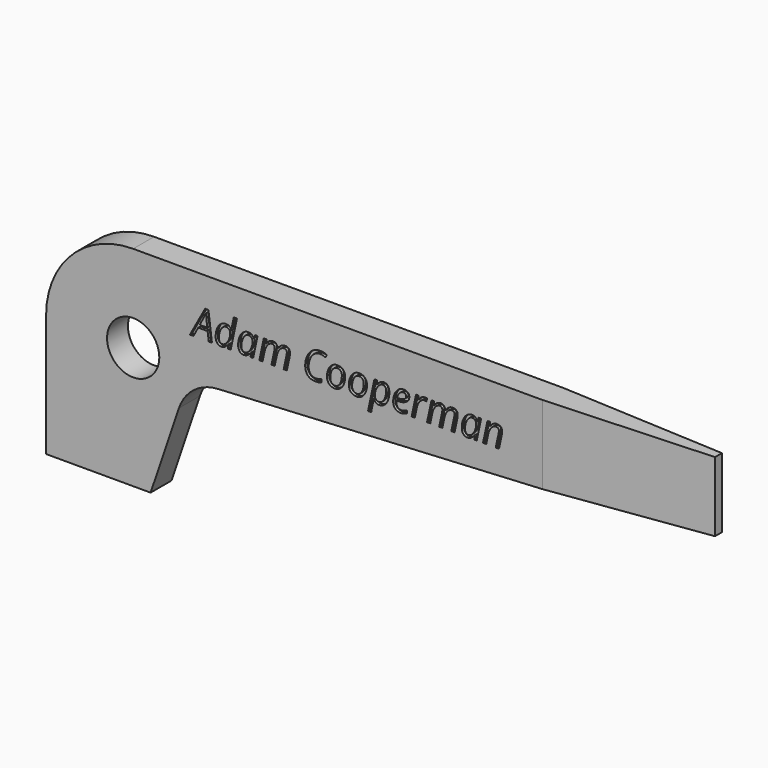
from build123d import *

# Parameters (mm, degrees)
F1_DEPTH     = 2.38125
F2_R         = 2.38125
F3_DEPTH     = 2.38225
F5_DEPTH     = 25.4
F6_TEXT_SIZE = 3.5491733191
F7_DEPTH     = 0.254


# Not quite as in the source:
# - Text() gives the source's letters only with a copy of the font that has no kerning and outlines rounded to 1/6400 em; it was checked with that copy


with BuildPart() as f1:
    # F0 (on Front) → F1 (new body)
    with BuildSketch(Plane.XZ):
        with BuildLine():
            Line((60.325, 19.05), (7.9375, 19.05))
            ThreePointArc((7.9375, 19.05), (2.3248399243, 16.7251600757), (0, 11.1125))
            Line((0, 11.1125), (0, 0))
            Line((0, 0), (9.525, 0))
            Line((9.525, 0), (12.1103451907, 7.6262422093))
            ThreePointArc((12.1103451907, 7.6262422093), (13.4737562991, 9.5178776332), (15.6634210502, 10.3194652484))
            Line((15.6634210502, 10.3194652484), (60.325, 12.7))
            Line((60.325, 12.7), (60.325, 19.05))
        make_face()
    extrude(amount=F1_DEPTH)

    # F2 (on face) → F3 (cut, through all)
    with BuildSketch(Plane.XZ.offset(2.38125)):
        with Locations((7.9375, 11.1125)):
            Circle(F2_R)
    extrude(amount=-F3_DEPTH, mode=Mode.SUBTRACT)

    # F4 (on face) → F5 (cut)
    with BuildSketch(Plane.XY.offset(19.05)):
        Polygon((60.325, -2.38125), (60.325, -1.5875), (45.2374, -2.38125), align=None)
        Polygon((60.325, 0), (45.2374, 0), (60.325, -0.79375), align=None)
    extrude(amount=-F5_DEPTH, mode=Mode.SUBTRACT)

    # F6 (on face) → F7 (cut)
    with BuildSketch(Plane.XZ.offset(2.38125)):
        with Locations((13.3138839155, 13.8433789834)):
            Text('Adam Cooperman', F6_TEXT_SIZE, font='Open Sans', font_style=FontStyle.ITALIC, text_align=(TextAlign.LEFT, TextAlign.BOTTOM))
    extrude(amount=-F7_DEPTH, mode=Mode.SUBTRACT)


solid = f1.part
